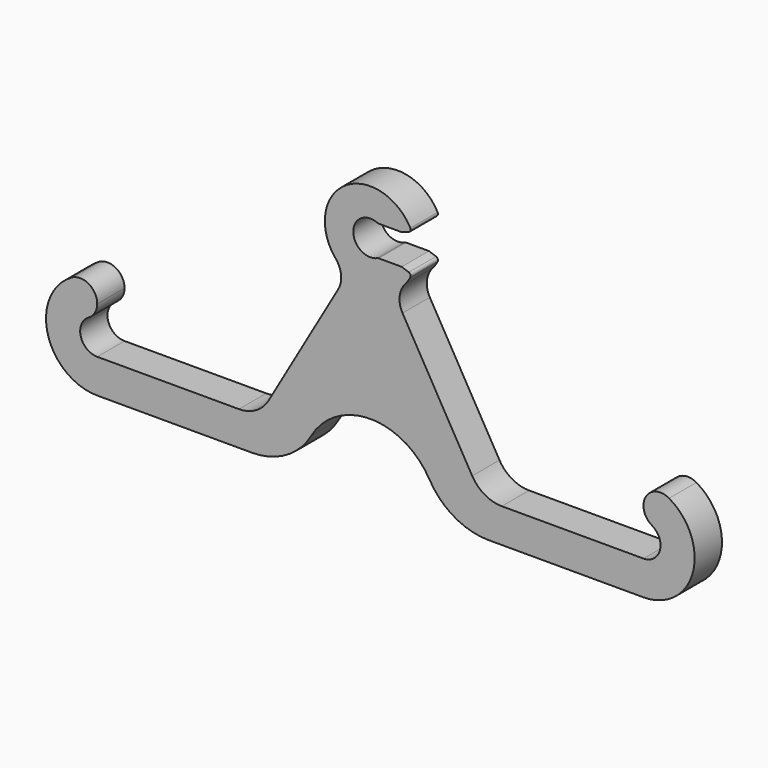
from build123d import *

# Parameters (mm, degrees)
F1_DEPTH    = 2.38125
F2_DEPTH    = 2.38125
F3_T1_DEPTH = 6.5449897521
F3_T3_DEPTH = 6.5449897521
F4_T1_DEPTH = 13.0899795043
F5_R        = 0.396875
F6_R        = 3.175
F7_R        = 2.38124
F9_DEPTH    = 4.7635
F10_R       = 9.52499


# Not quite as in the source:
# - a fillet or chamfer that OpenCascade refuses, or shapes differently, is made with other operations: its cross-section is extruded or revolved along the edge and cut away or added
# - a fillet or chamfer is up to 0.001 mm smaller than in the source, because OpenCascade refuses the exact size


with BuildPart() as f1:
    # F0 (on Front) → F1 (new body, symmetric)
    with BuildSketch(Plane.XZ):
        with BuildLine():
            ThreePointArc((-38.1, 14.2875), (-45.24375, 7.14375), (-38.1, 0))
            Line((-38.1, 0), (38.1, 0))
            ThreePointArc((38.1, 0), (45.24375, 7.14375), (38.1, 14.2875))
            Line((38.1, 14.2875), (38.1, 9.525))
            ThreePointArc((38.1, 9.525), (40.48125, 7.14375), (38.1, 4.7625))
            Line((38.1, 4.7625), (18.3308710468, 4.7625))
            ThreePointArc((18.3308710468, 4.7625), (15.9496210468, 5.4005540145), (14.2064250612, 7.14375))
            Line((14.2064250612, 7.14375), (3.175, 26.250738686))
            ThreePointArc((3.175, 26.250738686), (0, 25.4), (-3.175, 26.250738686))
            Line((-3.175, 26.250738686), (-14.2064250612, 7.14375))
            ThreePointArc((-14.2064250612, 7.14375), (-15.9496210468, 5.4005540145), (-18.3308710468, 4.7625))
            Line((-18.3308710468, 4.7625), (-38.1, 4.7625))
            ThreePointArc((-38.1, 4.7625), (-40.48125, 7.14375), (-38.1, 9.525))
            Line((-38.1, 9.525), (-38.1, 14.2875))
        make_face()
    extrude(amount=F1_DEPTH, both=True)

    # F0 (on Front) → F2 (join, symmetric)
    with BuildSketch(Plane.XZ):
        with BuildLine():
            ThreePointArc((5.9830851103, 33.87725), (-4.0635273104, 36.6295743459), (-3.175, 26.250738686))
            ThreePointArc((-3.175, 26.250738686), (0, 25.4), (3.175, 26.250738686))
            ThreePointArc((3.175, 26.250738686), (4.8795743459, 27.6864726896), (5.9830851103, 29.62275))
            Line((5.9830851103, 29.62275), (1.0701210212, 29.62275))
            ThreePointArc((1.0701210212, 29.62275), (-2.38125, 31.75), (1.0701210212, 33.87725))
            Line((1.0701210212, 33.87725), (5.9830851103, 33.87725))
        make_face()
    extrude(amount=F2_DEPTH, both=True)

    # F3: chamfer of 0.396875 x 1.5875 on 2 edges, made by hand

    # F3_s2 → F3_t1 (cut)
    with BuildSketch(Plane.XZ):
        with BuildLine():
            Line((5.8436173462, 34.3923519359), (4.3177222428, 33.8561996981))
            Line((4.3177222428, 33.8561996981), (4.3177222428, 33.8244496981))
            ThreePointArc((4.3177222428, 33.8244496981), (5.1504036766, 33.8455), (5.9830851103, 33.8455))
            Line((5.9830851103, 33.8455), (6.0130005359, 33.88788625))
            ThreePointArc((6.0130005359, 33.88788625), (5.918565904, 34.1369039994), (5.872535886, 34.405458444))
            Line((5.872535886, 34.405458444), (5.8436173462, 34.3923519359))
        make_face()
    extrude(amount=F3_T1_DEPTH, mode=Mode.SUBTRACT)

    # F3_s4 → F3_t3 (cut)
    with BuildSketch(Plane.XZ.offset(-6.5449897521)):
        with BuildLine():
            Line((5.8436173462, 34.3923519359), (4.3177222428, 33.8561996981))
            Line((4.3177222428, 33.8561996981), (4.3177222428, 33.8244496981))
            ThreePointArc((4.3177222428, 33.8244496981), (5.1504036766, 33.8455), (5.9830851103, 33.8455))
            Line((5.9830851103, 33.8455), (6.0130005359, 33.88788625))
            ThreePointArc((6.0130005359, 33.88788625), (5.918565904, 34.1369039994), (5.872535886, 34.405458444))
            Line((5.872535886, 34.405458444), (5.8436173462, 34.3923519359))
        make_face()
    extrude(amount=F3_T3_DEPTH, mode=Mode.SUBTRACT)

    # F4: chamfer of 1.5875 x 0.396875 on 1 edges, made by hand

    # F4_s2 → F4_t1 (cut)
    with BuildSketch(Plane.XZ.offset(-6.5449897521)):
        with BuildLine():
            Line((4.3177222428, 29.6438003019), (5.8436173462, 29.1076480641))
            Line((5.8436173462, 29.1076480641), (5.872535886, 29.094541556))
            ThreePointArc((5.872535886, 29.094541556), (5.918565904, 29.3630960006), (6.0130005359, 29.61211375))
            Line((6.0130005359, 29.61211375), (5.9830851103, 29.6545))
            ThreePointArc((5.9830851103, 29.6545), (5.1504036766, 29.6545), (4.3177222428, 29.6755503019))
            Line((4.3177222428, 29.6755503019), (4.3177222428, 29.6438003019))
        make_face()
    extrude(amount=F4_T1_DEPTH, mode=Mode.SUBTRACT)

    # F5
    f5_edges = [f1.edges().sort_by_distance(p)[0] for p in [
        (5.783708, 0, 34.371302),
        (5.783708, 0, 29.128698),
        (1.070121, 0, 29.62275),
        (1.070121, 0, 33.87725),
    ]]
    fillet(f5_edges, radius=F5_R)

    # F6
    f6_edges = [f1.edges().sort_by_distance(p)[0] for p in [
        (3.175, 0, 26.250739),
        (-3.175, 0, 26.250739),
    ]]
    fillet(f6_edges, radius=F6_R)

    # F7 (radius 2.38125 in the source; OpenCascade refuses exactly that, so slightly less here)
    f7_edges = [f1.edges().sort_by_distance(p)[0] for p in [
        (38.1, 0, 14.2875),
        (38.1, 0, 9.525),
        (-38.1, 0, 14.2875),
        (-38.1, 0, 9.525),
    ]]
    fillet(f7_edges, radius=F7_R)

    # F8 (on face) → F9 (cut, through all)
    with BuildSketch(Plane.XZ.offset(2.38125)):
        Polygon((10.9985226281, 0), (0, 19.05), (-10.9985226281, 0), align=None)
    extrude(amount=-F9_DEPTH, mode=Mode.SUBTRACT)

    # F10 (radius 9.525 in the source; OpenCascade refuses exactly that, so slightly less here)
    f10_edges = [f1.edges().sort_by_distance(p)[0] for p in [
        (0, 0, 19.05),
        (10.998523, 0, 0),
        (-10.998523, 0, 0),
    ]]
    fillet(f10_edges, radius=F10_R)


solid = f1.part
